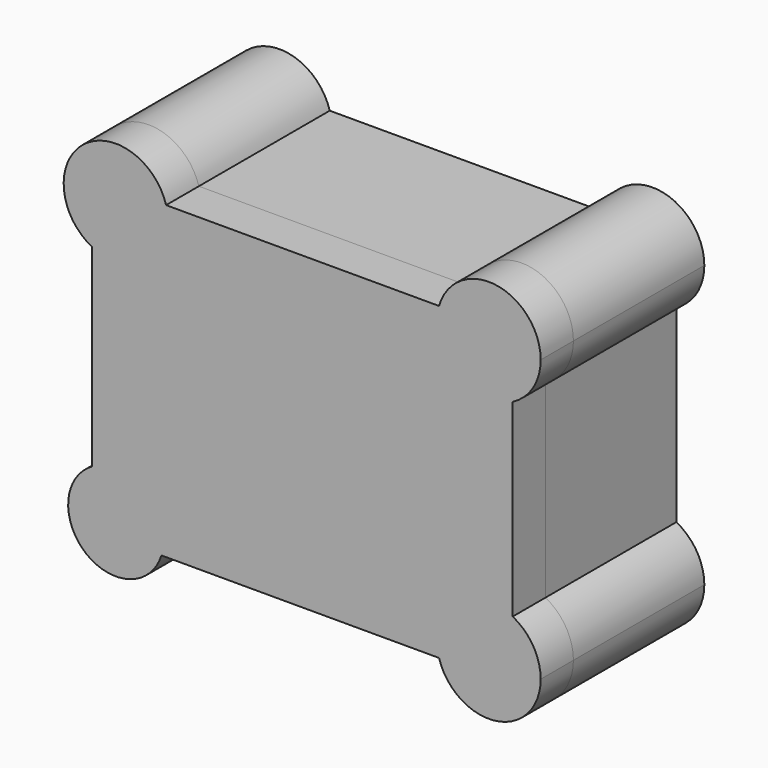
from build123d import *

# Parameters (mm, degrees)
F0_R     = 20.1212122489
F1_DEPTH = 31.75
F2_DEPTH = 25.4
F4_DEPTH = 25.4


with BuildPart() as f1:
    # F0 (on Front) → F1 (new body)
    with BuildSketch(Plane.XZ):
        with BuildLine():
            ThreePointArc((28.9441868663, 13.7714213436), (23.2555589405, 16.1277281818), (20.8992521023, 21.8163561076))
            Line((20.8992521023, 21.8163561076), (-20.8388379964, 21.8163561076))
            ThreePointArc((-20.8388379964, 21.8163561076), (-23.2128397165, 16.0850089578), (-28.9441868663, 13.7110072377))
            Line((-28.9441868663, 13.7110072377), (-28.9441868663, -14.408954399))
            ThreePointArc((-28.9441868663, -14.408954399), (-23.7063628872, -16.5785321285), (-21.5367851577, -21.8163561076))
            Line((-21.5367851577, -21.8163561076), (20.8992521023, -21.8163561076))
            ThreePointArc((20.8992521023, -21.8163561076), (23.2555589405, -16.1277281818), (28.9441868663, -13.7714213436))
            Line((28.9441868663, -13.7714213436), (28.9441868663, 13.7714213436))
        make_face()
        Circle(F0_R, mode=Mode.SUBTRACT)
        Circle(F0_R)
        with BuildLine():
            ThreePointArc((-28.9441868663, 13.7110072377), (-23.2128397165, 16.0850089578), (-20.8388379964, 21.8163561076))
            ThreePointArc((-20.8388379964, 21.8163561076), (-20.9175451076, 22.9431668192), (-21.1521378679, 24.0480937064))
            ThreePointArc((-21.1521378679, 24.0480937064), (-34.0896867071, 28.0789842852), (-32.6450914145, 14.6052545393))
            ThreePointArc((-32.6450914145, 14.6052545393), (-30.8478919847, 13.9377402949), (-28.9441868663, 13.7110072377))
        make_face()
        with BuildLine():
            ThreePointArc((21.2150004507, 24.0480937064), (20.9785803028, 22.9433376657), (20.8992521023, 21.8163561076))
            ThreePointArc((20.8992521023, 21.8163561076), (23.2555589405, 16.1277281818), (28.9441868663, 13.7714213436))
            ThreePointArc((28.9441868663, 13.7714213436), (30.8487832476, 14.0001237684), (32.6450914145, 14.6732278796))
            ThreePointArc((32.6450914145, 14.6732278796), (35.8178507733, 17.6361982339), (36.9891216302, 21.8163561076))
            ThreePointArc((36.9891216302, 21.8163561076), (30.0711684244, 29.7819626711), (21.2150004507, 24.0480937064))
        make_face()
        with BuildLine():
            ThreePointArc((32.6450914145, -14.6732278796), (30.8487832476, -14.0001237684), (28.9441868663, -13.7714213436))
            ThreePointArc((28.9441868663, -13.7714213436), (23.2555589405, -16.1277281818), (20.8992521023, -21.8163561076))
            ThreePointArc((20.8992521023, -21.8163561076), (20.9785803028, -22.9433376657), (21.2150004507, -24.0480937064))
            ThreePointArc((21.2150004507, -24.0480937064), (30.0711684244, -29.7819626711), (36.9891216302, -21.8163561076))
            ThreePointArc((36.9891216302, -21.8163561076), (35.8178507733, -17.6361982339), (32.6450914145, -14.6732278796))
        make_face()
        with BuildLine():
            ThreePointArc((-21.5367851577, -21.8163561076), (-23.7063628872, -16.5785321285), (-28.9441868663, -14.408954399))
            ThreePointArc((-28.9441868663, -14.408954399), (-30.8598042167, -14.6609378641), (-32.6450914145, -15.3997444162))
            ThreePointArc((-32.6450914145, -15.3997444162), (-33.5836655288, -27.5908550306), (-21.8809760268, -24.0480937064))
            ThreePointArc((-21.8809760268, -24.0480937064), (-21.6233385509, -22.9454176719), (-21.5367851577, -21.8163561076))
        make_face()
        with BuildLine():
            Line((-28.9441868663, -14.408954399), (-28.9441868663, 13.7110072377))
            ThreePointArc((-28.9441868663, 13.7110072377), (-30.8478919847, 13.9377402949), (-32.6450914145, 14.6052545393))
            Line((-32.6450914145, 14.6052545393), (-32.6450914145, -15.3997444162))
            ThreePointArc((-32.6450914145, -15.3997444162), (-30.8598042167, -14.6609378641), (-28.9441868663, -14.408954399))
        make_face()
        with BuildLine():
            ThreePointArc((32.6450914145, 14.6732278796), (30.8487832476, 14.0001237684), (28.9441868663, 13.7714213436))
            Line((28.9441868663, 13.7714213436), (28.9441868663, -13.7714213436))
            ThreePointArc((28.9441868663, -13.7714213436), (30.8487832476, -14.0001237684), (32.6450914145, -14.6732278796))
            Line((32.6450914145, -14.6732278796), (32.6450914145, 14.6732278796))
        make_face()
        with BuildLine():
            ThreePointArc((21.2150004507, -24.0480937064), (20.9785803028, -22.9433376657), (20.8992521023, -21.8163561076))
            Line((20.8992521023, -21.8163561076), (-21.5367851577, -21.8163561076))
            ThreePointArc((-21.5367851577, -21.8163561076), (-21.6233385509, -22.9454176719), (-21.8809760268, -24.0480937064))
            Line((-21.8809760268, -24.0480937064), (21.2150004507, -24.0480937064))
        make_face()
        with BuildLine():
            Line((-20.8388379964, 21.8163561076), (20.8992521023, 21.8163561076))
            ThreePointArc((20.8992521023, 21.8163561076), (20.9785803028, 22.9433376657), (21.2150004507, 24.0480937064))
            Line((21.2150004507, 24.0480937064), (-21.1521378679, 24.0480937064))
            ThreePointArc((-21.1521378679, 24.0480937064), (-20.9175451076, 22.9431668192), (-20.8388379964, 21.8163561076))
        make_face()
    extrude(amount=F1_DEPTH)


with BuildPart() as f2:
    # F0 (on Front) → F2 (new body)
    with BuildSketch(Plane.XZ):
        with BuildLine():
            Line((-20.8388379964, 21.8163561076), (20.8992521023, 21.8163561076))
            ThreePointArc((20.8992521023, 21.8163561076), (20.9785803028, 22.9433376657), (21.2150004507, 24.0480937064))
            Line((21.2150004507, 24.0480937064), (-21.1521378679, 24.0480937064))
            ThreePointArc((-21.1521378679, 24.0480937064), (-20.9175451076, 22.9431668192), (-20.8388379964, 21.8163561076))
        make_face()
        with BuildLine():
            ThreePointArc((21.2150004507, 24.0480937064), (20.9785803028, 22.9433376657), (20.8992521023, 21.8163561076))
            ThreePointArc((20.8992521023, 21.8163561076), (23.2555589405, 16.1277281818), (28.9441868663, 13.7714213436))
            ThreePointArc((28.9441868663, 13.7714213436), (30.8487832476, 14.0001237684), (32.6450914145, 14.6732278796))
            ThreePointArc((32.6450914145, 14.6732278796), (35.8178507733, 17.6361982339), (36.9891216302, 21.8163561076))
            ThreePointArc((36.9891216302, 21.8163561076), (30.0711684244, 29.7819626711), (21.2150004507, 24.0480937064))
        make_face()
        with BuildLine():
            ThreePointArc((-28.9441868663, 13.7110072377), (-23.2128397165, 16.0850089578), (-20.8388379964, 21.8163561076))
            ThreePointArc((-20.8388379964, 21.8163561076), (-20.9175451076, 22.9431668192), (-21.1521378679, 24.0480937064))
            ThreePointArc((-21.1521378679, 24.0480937064), (-34.0896867071, 28.0789842852), (-32.6450914145, 14.6052545393))
            ThreePointArc((-32.6450914145, 14.6052545393), (-30.8478919847, 13.9377402949), (-28.9441868663, 13.7110072377))
        make_face()
        with BuildLine():
            ThreePointArc((32.6450914145, 14.6732278796), (30.8487832476, 14.0001237684), (28.9441868663, 13.7714213436))
            Line((28.9441868663, 13.7714213436), (28.9441868663, -13.7714213436))
            ThreePointArc((28.9441868663, -13.7714213436), (30.8487832476, -14.0001237684), (32.6450914145, -14.6732278796))
            Line((32.6450914145, -14.6732278796), (32.6450914145, 14.6732278796))
        make_face()
        with BuildLine():
            Line((-28.9441868663, -14.408954399), (-28.9441868663, 13.7110072377))
            ThreePointArc((-28.9441868663, 13.7110072377), (-30.8478919847, 13.9377402949), (-32.6450914145, 14.6052545393))
            Line((-32.6450914145, 14.6052545393), (-32.6450914145, -15.3997444162))
            ThreePointArc((-32.6450914145, -15.3997444162), (-30.8598042167, -14.6609378641), (-28.9441868663, -14.408954399))
        make_face()
        with BuildLine():
            ThreePointArc((32.6450914145, -14.6732278796), (30.8487832476, -14.0001237684), (28.9441868663, -13.7714213436))
            ThreePointArc((28.9441868663, -13.7714213436), (23.2555589405, -16.1277281818), (20.8992521023, -21.8163561076))
            ThreePointArc((20.8992521023, -21.8163561076), (20.9785803028, -22.9433376657), (21.2150004507, -24.0480937064))
            ThreePointArc((21.2150004507, -24.0480937064), (30.0711684244, -29.7819626711), (36.9891216302, -21.8163561076))
            ThreePointArc((36.9891216302, -21.8163561076), (35.8178507733, -17.6361982339), (32.6450914145, -14.6732278796))
        make_face()
        with BuildLine():
            ThreePointArc((-21.5367851577, -21.8163561076), (-23.7063628872, -16.5785321285), (-28.9441868663, -14.408954399))
            ThreePointArc((-28.9441868663, -14.408954399), (-30.8598042167, -14.6609378641), (-32.6450914145, -15.3997444162))
            ThreePointArc((-32.6450914145, -15.3997444162), (-33.5836655288, -27.5908550306), (-21.8809760268, -24.0480937064))
            ThreePointArc((-21.8809760268, -24.0480937064), (-21.6233385509, -22.9454176719), (-21.5367851577, -21.8163561076))
        make_face()
        with BuildLine():
            ThreePointArc((21.2150004507, -24.0480937064), (20.9785803028, -22.9433376657), (20.8992521023, -21.8163561076))
            Line((20.8992521023, -21.8163561076), (-21.5367851577, -21.8163561076))
            ThreePointArc((-21.5367851577, -21.8163561076), (-21.6233385509, -22.9454176719), (-21.8809760268, -24.0480937064))
            Line((-21.8809760268, -24.0480937064), (21.2150004507, -24.0480937064))
        make_face()
    extrude(amount=F2_DEPTH)

    # F3 (on face) → F4 (cut)
    with BuildSketch(Plane(origin=(0, 0, -24.0480937064), x_dir=(1, 0, 0), z_dir=(0, 0, -1))):
        with BuildLine():
            Line((-5.5820932612, 8.2697672769), (-5.5820932612, 0))
            Line((-5.5820932612, 0), (3.3079062123, 0))
            Line((3.3079062123, 0), (3.3079062123, 8.2697672769))
            ThreePointArc((3.3079062123, 8.2697672769), (-1.1370935244, 12.7147670137), (-5.5820932612, 8.2697672769))
        make_face()
    extrude(amount=-F4_DEPTH, mode=Mode.SUBTRACT)


with BuildPart() as f2b:
    # F0 (on Front) → F2, piece 2 (new body)
    with BuildSketch(Plane.XZ):
        Circle(F0_R)
    extrude(amount=F2_DEPTH)


solid = Compound([f1.part, f2.part, f2b.part])
